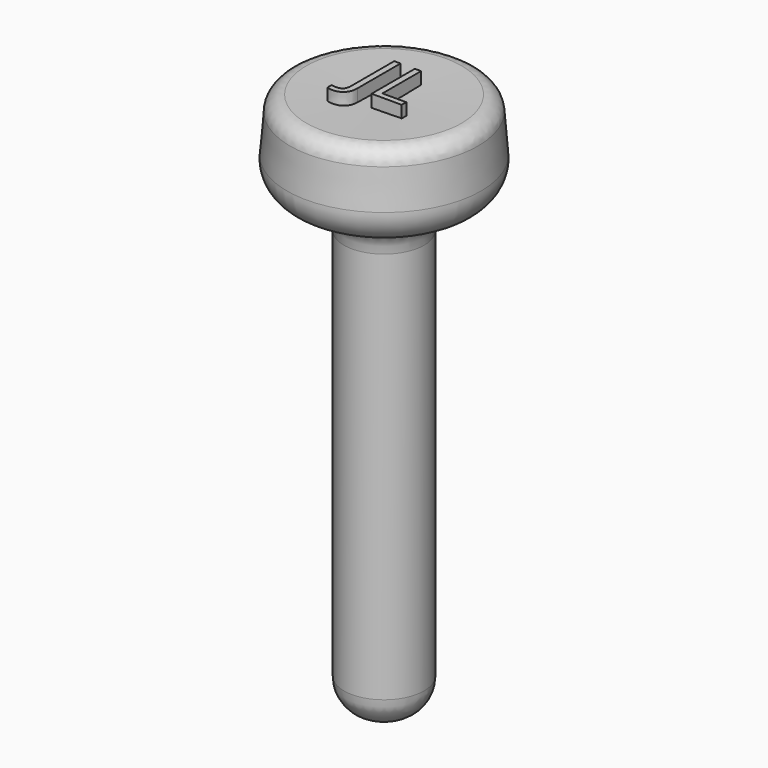
from build123d import *

# Parameters (mm, degrees)
F2_R         = 5.08
F3_R         = 5.08
F4_R         = 2.54
F5_R         = 5.08
F6_TEXT_SIZE = 11.9747548726
F7_DEPTH     = 2.032


# Not quite as in the source:
# - Text() gives the source's letters only with a copy of the font that has no kerning and outlines rounded to 1/6400 em; it was checked with that copy


with BuildPart() as f1:
    # F0 (on Front) → F1 (revolve)
    with BuildSketch(Plane.XZ):
        with BuildLine():
            ThreePointArc((0, -35.3421096606), (3.3779014502, -34.7413555039), (6.3415337354, -33.0127701163))
            Line((6.3415337354, -33.0127701163), (6.3415337354, 37.0202325284))
            Line((6.3415337354, 37.0202325284), (15.8123914152, 37.0202325284))
            Line((15.8123914152, 37.0202325284), (14.6947761936, 51.0076284409))
            Line((14.6947761936, 51.0076284409), (0.5310886315, 50.6729638469))
            Line((0.5310886315, 50.6729638469), (0, 50.6729638469))
            Line((0, 50.6729638469), (0, -25.5451539221))
            Line((0, -25.5451539221), (0, -35.3421096606))
        make_face()
    revolve(axis=Axis((0, 0, 20.0786253562), (0, 0, 1)))

    # F2
    f2_edges = [f1.edges().sort_by_distance(p)[0] for p in [
        (-15.812391, 0, 37.020233),
    ]]
    fillet(f2_edges, radius=F2_R)

    # F3
    f3_edges = [f1.edges().sort_by_distance(p)[0] for p in [
        (-6.341534, 0, -33.01277),
    ]]
    fillet(f3_edges, radius=F3_R)

    # F4
    f4_edges = [f1.edges().sort_by_distance(p)[0] for p in [
        (-14.694776, 0, 51.007628),
    ]]
    fillet(f4_edges, radius=F4_R)

    # F5
    f5_edges = [f1.edges().sort_by_distance(p)[0] for p in [
        (-6.341534, 0, 37.020233),
    ]]
    fillet(f5_edges, radius=F5_R)

    # F6 (on face) → F7 (join)
    with BuildSketch(Plane.XY.offset(50.6729638469)):
        with Locations((-3.5975568462, -3.4283720888)):
            Text('JL', F6_TEXT_SIZE, font='Open Sans', text_align=(TextAlign.LEFT, TextAlign.BOTTOM))
    extrude(amount=F7_DEPTH)


solid = f1.part
